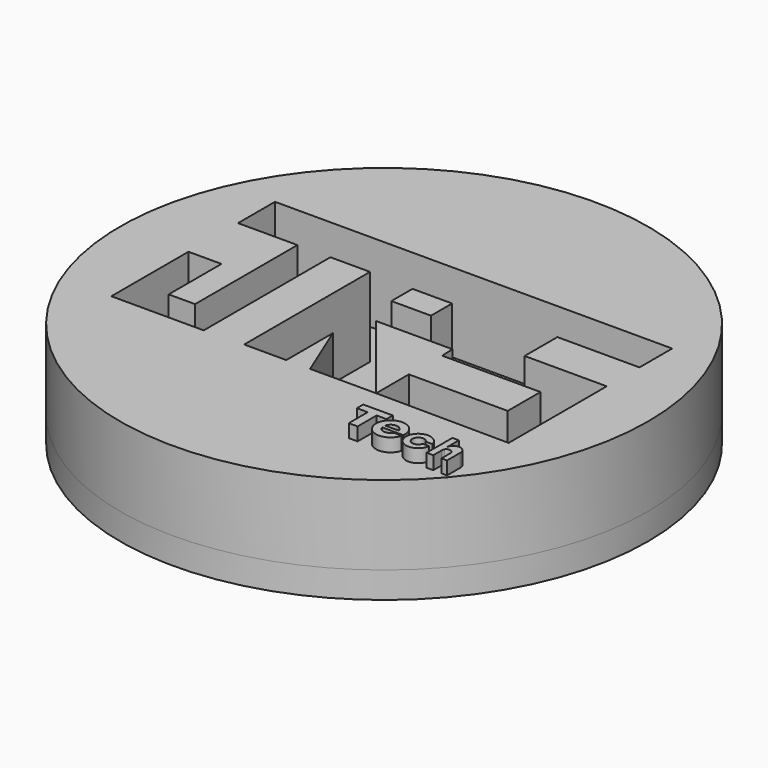
from build123d import *

# Parameters (mm, degrees)
F0_R     = 20
F1_DEPTH = 6
F0_W     = 3
F0_H     = 2
F2_DEPTH = 6
F3_DEPTH = 6
F6_R     = 20
F7_DEPTH = 2
F9_DEPTH = 1


# Not quite as in the source:
# - the program builds the solid bodies; features that only make, move or delete a surface that nothing else refers to are left out


with BuildPart() as f1:
    # F0 (on Top) → F1 (new body)
    with BuildSketch(Plane.XY):
        Circle(F0_R)
        Polygon((-14.8229663414, 4.6952926321), (-14.8229663414, 8.1952926321), (-4.8229663414, 8.1952926321), (5.1770336586, 8.1952926321), (15.2737221277, 8.1952926321), (15.2737221277, 5.0952926321), (9.0523306343, 5.0952926321), (9.0523306343, 1.9952926321), (15.2737221277, 1.9952926321), (15.2737221277, -7.2968558197), (5.1770336586, -7.2245139418), (0.1770336586, -7.2245139418), (-1.6315090997, -2.8116659632), (-1.6315090997, -7.2245139418), (-4.8229663414, -7.2245139418), (-4.8229663414, 4.6952926321), (-7.8229663414, 4.6952926321), (-7.8229663414, -7.3047073679), (-14.8229663414, -7.3047073679), (-14.8229663414, 0), (-12.3229663414, 0), (-12.3229663414, -4.9991512411), (-10.3229663414, -4.9991512411), (-10.3229663414, 4.6952926321), align=None, mode=Mode.SUBTRACT)
    extrude(amount=F1_DEPTH)

    # F8 (on face) → F9 (join)
    with BuildSketch(Plane.XY.offset(6)):
        with BuildLine():
            Line((15.0292580947, -12.8243761654), (15.0292580947, -11.5819023922))
            ThreePointArc((15.0292580947, -11.5819023922), (14.9037661569, -11.9053522282), (14.6068680189, -12.0848501905))
            Line((14.6068680189, -12.0848501905), (14.6068680189, -12.8243761654))
            Line((14.6068680189, -12.8243761654), (15.0292580947, -12.8243761654))
        make_face()
        with BuildLine():
            ThreePointArc((15.0297242951, -11.5595152602), (14.5479652061, -11.0246856664), (13.965879567, -11.4481367533))
            ThreePointArc((13.965879567, -11.4481367533), (13.9595626035, -11.63513708), (14.0177011696, -11.8129823311))
            ThreePointArc((14.0177011696, -11.8129823311), (14.373767478, -11.6682234447), (14.6070883482, -11.9736734778))
            ThreePointArc((14.6070883482, -11.9736734778), (14.6070332611, -11.9795792393), (14.6068680189, -11.9854829456))
            Line((14.6068680189, -11.9854829456), (14.6068680189, -12.0848501905))
            ThreePointArc((14.6068680189, -12.0848501905), (14.9037661569, -11.9053522282), (15.0292580947, -11.5819023922))
            ThreePointArc((15.0292580947, -11.5819023922), (15.0296077324, -11.570711253), (15.0297242951, -11.5595152602))
        make_face()
        with BuildLine():
            Line((13.965879567, -10.3730093688), (13.4733673185, -10.3730093688))
            Line((13.4733673185, -10.3730093688), (13.4733673185, -12.8131825477))
            Line((13.4733673185, -12.8131825477), (13.977073133, -12.8131825477))
            Line((13.977073133, -12.8131825477), (13.977073133, -12.0184542606))
            ThreePointArc((13.977073133, -12.0184542606), (13.9799034833, -11.912261244), (14.0177011696, -11.8129823311))
            ThreePointArc((14.0177011696, -11.8129823311), (13.9595626035, -11.63513708), (13.965879567, -11.4481367533))
            Line((13.965879567, -11.4481367533), (13.965879567, -10.3730093688))
        make_face()
        with BuildLine():
            Line((12.5385226393, -11.7363042429), (13.0446804071, -11.7363042429))
            ThreePointArc((13.0446804071, -11.7363042429), (11.2134738953, -11.990157639), (13.0611900744, -12.0510161396))
            Line((13.0611900744, -12.0510161396), (12.5746978874, -12.0510161396))
            ThreePointArc((12.5746978874, -12.0510161396), (11.6945373163, -11.992753054), (12.5385226393, -11.7363042429))
        make_face()
        with BuildLine():
            Line((10.4112224445, -11.6244971905), (10.9858511253, -11.6244971905))
            ThreePointArc((10.9858511253, -11.6244971905), (8.7959122239, -11.6808773259), (10.9590917495, -12.0268042712))
            Line((10.9590917495, -12.0268042712), (10.352076243, -12.0268042712))
            ThreePointArc((10.352076243, -12.0268042712), (9.8306001316, -12.2838217189), (9.3837593923, -11.9118961121))
            ThreePointArc((9.3837593923, -11.9118961121), (9.3600362793, -11.7687460957), (9.3757514516, -11.6244971905))
            ThreePointArc((9.3757514516, -11.6244971905), (9.893486948, -11.2202245839), (10.4112224445, -11.6244971905))
        make_face()
        with BuildLine():
            ThreePointArc((10.9820785301, -11.9118961121), (10.9906311364, -11.8330948527), (10.993486948, -11.7538822913))
            ThreePointArc((10.993486948, -11.7538822913), (10.9915763331, -11.6890771794), (10.9858511253, -11.6244971905))
            Line((10.9858511253, -11.6244971905), (10.4112224445, -11.6244971905))
            ThreePointArc((10.4112224445, -11.6244971905), (10.4231491454, -11.6887017322), (10.4271446554, -11.7538822913))
            ThreePointArc((10.4271446554, -11.7538822913), (10.4211282028, -11.8337900814), (10.4032145037, -11.9118961121))
            Line((10.4032145037, -11.9118961121), (10.9820785301, -11.9118961121))
        make_face()
        with BuildLine():
            ThreePointArc((10.4271446554, -11.7538822913), (10.4231491454, -11.6887017322), (10.4112224445, -11.6244971905))
            Line((10.4112224445, -11.6244971905), (9.3757514516, -11.6244971905))
            ThreePointArc((9.3757514516, -11.6244971905), (9.3600362793, -11.7687460957), (9.3837593923, -11.9118961121))
            Line((9.3837593923, -11.9118961121), (10.4032145037, -11.9118961121))
            ThreePointArc((10.4032145037, -11.9118961121), (10.4211282028, -11.8337900814), (10.4271446554, -11.7538822913))
        make_face()
        Polygon((8.9217557242, -10.3269937025), (6.6808465031, -10.3269937025), (6.6808465031, -10.9269937025), (7.5050893758, -10.9269937025), (7.5050893758, -12.7269937025), (8.1747866203, -12.7269937025), (8.1747866203, -10.9269937025), (8.9217557242, -10.9269937025), align=None)
    extrude(amount=F9_DEPTH)


with BuildPart() as f2:
    # F0 (on Top) → F2 (new body)
    with BuildSketch(Plane.XY):
        with Locations((0, 3.5671954031)):
            Rectangle(F0_W, F0_H)
    extrude(amount=F2_DEPTH)


with BuildPart() as f3:
    # F0 (on Top) → F3 (new body)
    with BuildSketch(Plane.XY):
        Polygon((5.2182162243, -1.0245139418), (5.1770336586, 0), (-0.6229663414, 0), (5.1770336586, -7.2245139418), (5.1770336586, -4.1245139418), (12.6694194104, -4.1245139418), (12.6694194104, -1.0245139418), align=None)
    extrude(amount=F3_DEPTH)


with BuildPart() as f7:
    # F6 (on face) → F7 (new body)
    with BuildSketch(Plane.XY):
        Circle(F6_R)
    extrude(amount=-F7_DEPTH)


solid = Compound([f1.part, f2.part, f3.part, f7.part])
